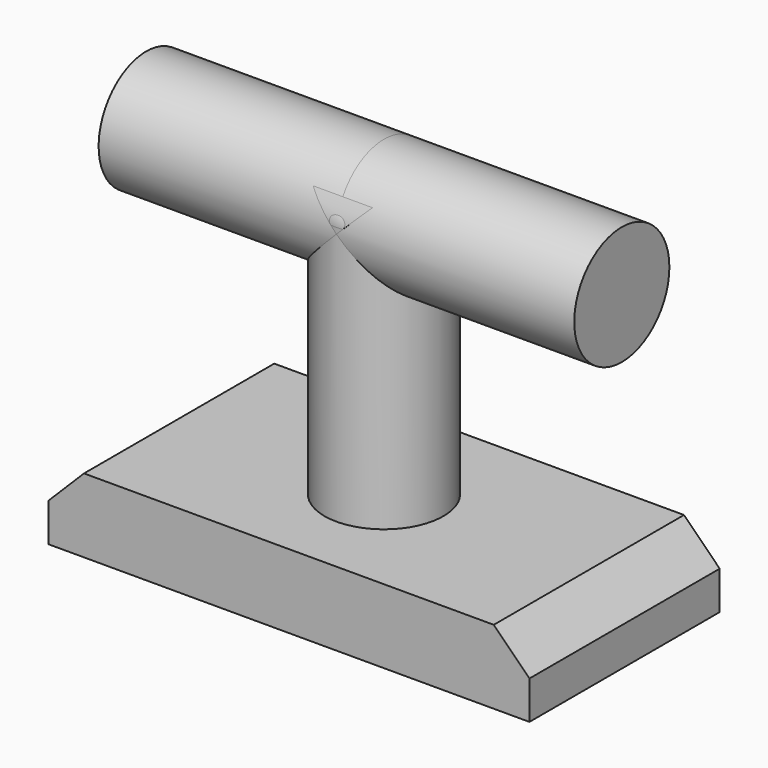
from build123d import *

# Parameters (mm, degrees)
F0_W         = 12.7
F0_H         = 6.35
F0_H_2       = 47.7120632529
F0_H_3       = 15.7879367471
F0_W_2       = 38.6885356486
F2_DEPTH     = 25.4
F4_DEPTH     = 50.8
F5_SIZE      = 7.62
F6_T4_ANGLE  = 174.612014659
F6_S5_R      = 12.7
F6_T6_DEPTH  = 17
F6_T10_ANGLE = 174.612014659
F6_S11_R     = 12.7
F6_T12_DEPTH = 17


# Not quite as in the source:
# - a fillet or chamfer that OpenCascade refuses, or shapes differently, is made with other operations: its cross-section is extruded or revolved along the edge and cut away or added


with BuildPart() as f1:
    # F0 (on Front) → F1 (revolve)
    with BuildSketch(Plane.XZ):
        with Locations((-6.35, 73.025)):
            Rectangle(F0_W, F0_H)
        with Locations((-6.35, 66.675)):
            Rectangle(F0_W, F0_H)
        with Locations((-6.35, 39.6439683735)):
            Rectangle(F0_W, F0_H_2)
    revolve(axis=Axis((0, 0, 38.1), (0, 0, 1)))

    # F0 (on Front) → F2 (join, symmetric)
    with BuildSketch(Plane.XZ):
        with Locations((-6.35, 7.8939683735)):
            Rectangle(F0_W, F0_H_3)
        with Locations((6.35, 7.8939683735)):
            Rectangle(F0_W, F0_H_3)
        with Locations((-32.0442678243, 7.8939683735)):
            Rectangle(F0_W_2, F0_H_3)
        with Locations((32.0442678243, 7.8939683735)):
            Rectangle(F0_W_2, F0_H_3)
    extrude(amount=F2_DEPTH, both=True)

    # F3 (on Right) → F4 (join, symmetric)
    with BuildSketch(Plane.YZ):
        with BuildLine():
            ThreePointArc((0, 57.15), (8.9802561211, 60.8697438789), (12.7, 69.85))
            ThreePointArc((12.7, 69.85), (-8.9802561211, 78.8302561211), (0, 57.15))
        make_face()
    extrude(amount=F4_DEPTH, both=True)

    # F5
    f5_edges = [f1.edges().sort_by_distance(p)[0] for p in [
        (-51.388536, 0, 15.787937),
        (51.388536, 0, 15.787937),
    ]]
    chamfer(f5_edges, length=F5_SIZE)

    # F6: fillet of radius 5.08 on 3 edges, made by hand


with BuildPart() as f6_tool2:
    # F6_s3 → F6_t4 (revolve)
    with BuildSketch(Plane(origin=(0, 0, 0), x_dir=(0, 0, 1), z_dir=(0.0470017192, -0.9988948085, 0))):
        with BuildLine():
            ThreePointArc((71.12, -12.7), (74.7121024484, -11.2121024484), (76.2, -7.62))
            Line((76.2, -7.62), (76.2, -12.7))
            Line((76.2, -12.7), (71.12, -12.7))
        make_face()
    revolve(axis=Axis((0, 0, 76.2), (0, 0, 1)), revolution_arc=F6_T4_ANGLE)

    # F6_s5 → F6_t6 (cut, symmetric)
    with BuildSketch(Plane.YZ):
        with Locations((0, 69.85)):
            Circle(F6_S5_R)
    extrude(amount=F6_T6_DEPTH, both=True, mode=Mode.SUBTRACT)


with BuildPart() as f1_1:
    add(f1.part)

    # F6_t1: cut F6_tool2
    add(f6_tool2.part, mode=Mode.SUBTRACT)


with BuildPart() as f6_tool8:
    # F6_s9 → F6_t10 (revolve)
    with BuildSketch(Plane(origin=(0, 0, 0), x_dir=(0, 0, 1), z_dir=(-0.0470017192, 0.9988948085, 0))):
        with BuildLine():
            ThreePointArc((71.12, -12.7), (74.7121024484, -11.2121024484), (76.2, -7.62))
            Line((76.2, -7.62), (76.2, -12.7))
            Line((76.2, -12.7), (71.12, -12.7))
        make_face()
    revolve(axis=Axis((0, 0, 76.2), (0, 0, 1)), revolution_arc=F6_T10_ANGLE)

    # F6_s11 → F6_t12 (cut, symmetric)
    with BuildSketch(Plane.YZ):
        with Locations((0, 69.85)):
            Circle(F6_S11_R)
    extrude(amount=F6_T12_DEPTH, both=True, mode=Mode.SUBTRACT)


with BuildPart() as f1_2:
    add(f1_1.part)

    # F6_t7: cut F6_tool8
    add(f6_tool8.part, mode=Mode.SUBTRACT)


solid = f1_2.part
